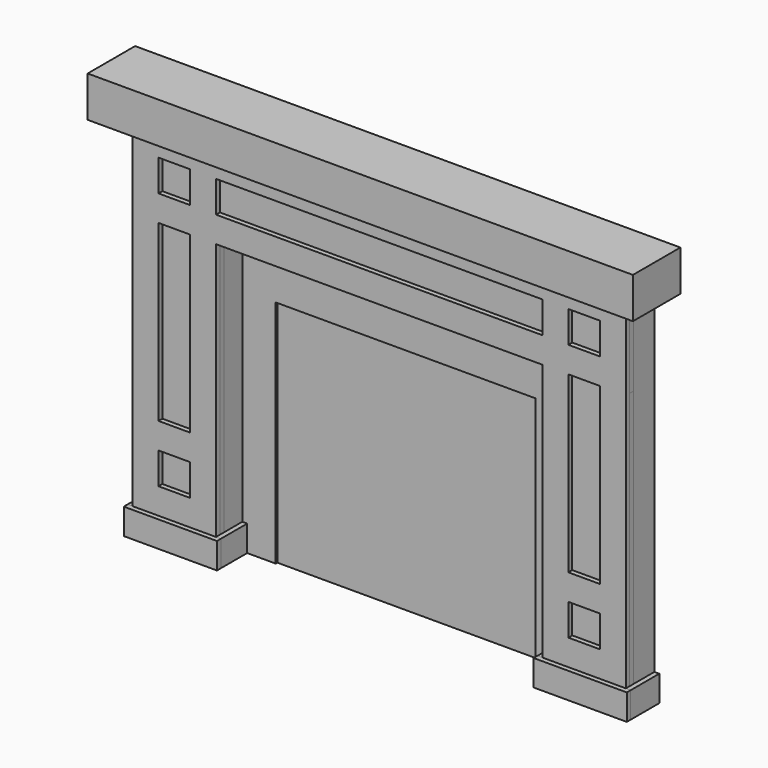
from build123d import *

# Parameters (mm, degrees)
F0_W      = 889
F0_H      = 787.4
F1_DEPTH  = 2.54
F3_DEPTH  = 9.525
F4_W      = 16.6624
F4_H      = 1240.6376
F5_DEPTH  = 88.9
F6_W      = 1689.1
F6_H      = 285.75
F7_DEPTH  = 16.6624
F8_W      = 285.75
F8_H      = 971.55
F9_DEPTH  = 16.6624
F10_W     = 107.95
F10_H     = 107.95
F10_H_2   = 596.9
F10_W_2   = 1117.6
F11_DEPTH = 16.6624
F12_W     = 319.0748
F12_H     = 88.9
F13_DEPTH = 16.6624
F15_DEPTH = 203.2
F16_W     = 122.2248
F16_H     = 88.9
F17_DEPTH = 16.6624
F18_W     = 105.5624
F18_H     = 88.9
F18_W_2   = 16.6624
F19_DEPTH = 16.6624
F20_W     = 16.6624
F20_H     = 971.55
F21_DEPTH = 79.375
F22_W     = 112.6998
F22_H     = 88.9
F23_DEPTH = 16.6624
F24_W     = 79.375
F24_H     = 88.9
F24_W_2   = 33.3248
F25_DEPTH = 16.6624


# Not quite as in the source:
# - a feature names something its author has since deleted; it is built from what else it names


with BuildPart() as f1:
    # F0 (on Front) → F1 (new body)
    with BuildSketch(Plane.XZ):
        with Locations((444.5, 393.7)):
            Rectangle(F0_W, F0_H)
    extrude(amount=F1_DEPTH)

    # F2 (on Front) → F3 (join)
    with BuildSketch(Plane.XZ):
        Polygon((-228.6, 0), (0, 0), (0, 787.4), (889, 787.4), (889, 0), (1117.6, 0), (1117.6, 1117.6), (-228.6, 1117.6), align=None)
    extrude(amount=F3_DEPTH)


with BuildPart() as f5:
    # F4 (on Front) → F5 (new body)
    with BuildSketch(Plane.XZ):
        with Locations((-391.7188, 620.3188)):
            Rectangle(F4_W, F4_H)
        Polygon((-383.3876, 1240.6376), (1272.3876, 1240.6376), (1289.05, 1240.6376), (1289.05, 1257.3), (-400.05, 1257.3), (-400.05, 1240.6376), align=None)
        with Locations((1280.7188, 620.3188)):
            Rectangle(F4_W, F4_H)
    extrude(amount=F5_DEPTH)


with BuildPart() as f7:
    # F6 (on face) → F7 (new body)
    with BuildSketch(Plane.XZ.offset(88.9)):
        with Locations((444.5, 1114.425)):
            Rectangle(F6_W, F6_H)
    extrude(amount=F7_DEPTH)


with BuildPart() as f9:
    # F8 (on face) → F9 (new body)
    with BuildSketch(Plane.XZ.offset(88.9)):
        with Locations((-257.175, 485.775)):
            Rectangle(F8_W, F8_H)
    extrude(amount=F9_DEPTH)


with BuildPart() as f9b:
    # F8 (on face) → F9, piece 2 (new body)
    with BuildSketch(Plane.XZ.offset(88.9)):
        with Locations((1146.175, 485.775)):
            Rectangle(F8_W, F8_H)
    extrude(amount=F9_DEPTH)


with BuildPart() as f11:
    # F10 (on face) → F11 (new body)
    with BuildSketch(Plane.XZ.offset(105.5624)):
        Polygon((-400.05, 971.55), (-400.05, 0), (-114.3, 0), (-114.3, 971.55), (1003.3, 971.55), (1003.3, 0), (1289.05, 0), (1289.05, 971.55), (1289.05, 1257.3), (-400.05, 1257.3), align=None)
        with Locations((-257.175, 231.775)):
            Rectangle(F10_W, F10_H, mode=Mode.SUBTRACT)
        with Locations((1146.175, 231.775)):
            Rectangle(F10_W, F10_H, mode=Mode.SUBTRACT)
        with Locations((-257.175, 673.1)):
            Rectangle(F10_W, F10_H_2, mode=Mode.SUBTRACT)
        with Locations((-257.175, 1114.425)):
            Rectangle(F10_W, F10_H, mode=Mode.SUBTRACT)
        with Locations((1146.175, 673.1)):
            Rectangle(F10_W, F10_H_2, mode=Mode.SUBTRACT)
        with Locations((444.5, 1114.425)):
            Rectangle(F10_W_2, F10_H, mode=Mode.SUBTRACT)
        with Locations((1146.175, 1114.425)):
            Rectangle(F10_W, F10_H, mode=Mode.SUBTRACT)
    extrude(amount=F11_DEPTH)

    # F12 (on face) → F13 (join)
    with BuildSketch(Plane.XZ.offset(122.2248)):
        with Locations((-257.175, 44.45)):
            Rectangle(F12_W, F12_H)
        with Locations((1146.175, 44.45)):
            Rectangle(F12_W, F12_H)
    extrude(amount=F13_DEPTH)


with BuildPart() as f15:
    # F14 (on Front) → F15 (new body)
    with BuildSketch(Plane.XZ):
        Polygon((-488.95, 1257.3), (-400.05, 1257.3), (1289.05, 1257.3), (1377.95, 1257.3), (1377.95, 1397), (-488.95, 1397), align=None)
    extrude(amount=F15_DEPTH)


with BuildPart() as f17:
    # F16 (on face) → F17 (new body)
    with BuildSketch(Plane.YZ.offset(1289.05)):
        with Locations((-61.1124, 44.45)):
            Rectangle(F16_W, F16_H)
    extrude(amount=F17_DEPTH)


with BuildPart() as f19:
    # F18 (on face) → F19 (new body)
    with BuildSketch(Plane(origin=(-400.05, 0, 0), x_dir=(0, -1, 0), z_dir=(-1, 0, 0))):
        with Locations((52.7812, 44.45)):
            Rectangle(F18_W, F18_H)
        with Locations((113.8936, 44.45)):
            Rectangle(F18_W_2, F18_H)
    extrude(amount=F19_DEPTH)


with BuildPart() as f21:
    # F20 (on face) → F21 (new body)
    with BuildSketch(Plane(origin=(0, -88.9, 0), x_dir=(-1, 0, 0), z_dir=(0, 1, 0))):
        with Locations((122.6312, 485.775)):
            Rectangle(F20_W, F20_H)
        Polygon((-1003.3, 971.55), (114.3, 971.55), (130.9624, 971.55), (130.9624, 988.2124), (-1019.9624, 988.2124), (-1019.9624, 971.55), align=None)
        with Locations((-1011.6312, 485.775)):
            Rectangle(F20_W, F20_H)
    extrude(amount=F21_DEPTH)


with BuildPart() as f23:
    # F22 (on face) → F23 (new body)
    with BuildSketch(Plane.YZ.offset(-114.3)):
        with Locations((-65.8749, 44.45)):
            Rectangle(F22_W, F22_H)
    extrude(amount=F23_DEPTH)


with BuildPart() as f25:
    # F24 (on face) → F25 (new body)
    with BuildSketch(Plane(origin=(1003.3, 0, 0), x_dir=(0, -1, 0), z_dir=(-1, 0, 0))):
        with Locations((49.2125, 44.45)):
            Rectangle(F24_W, F24_H)
        with Locations((105.5624, 44.45)):
            Rectangle(F24_W_2, F24_H)
    extrude(amount=F25_DEPTH)


solid = Compound([f1.part, f5.part, f7.part, f9.part, f9b.part, f11.part, f15.part, f17.part, f19.part, f21.part, f23.part, f25.part])
